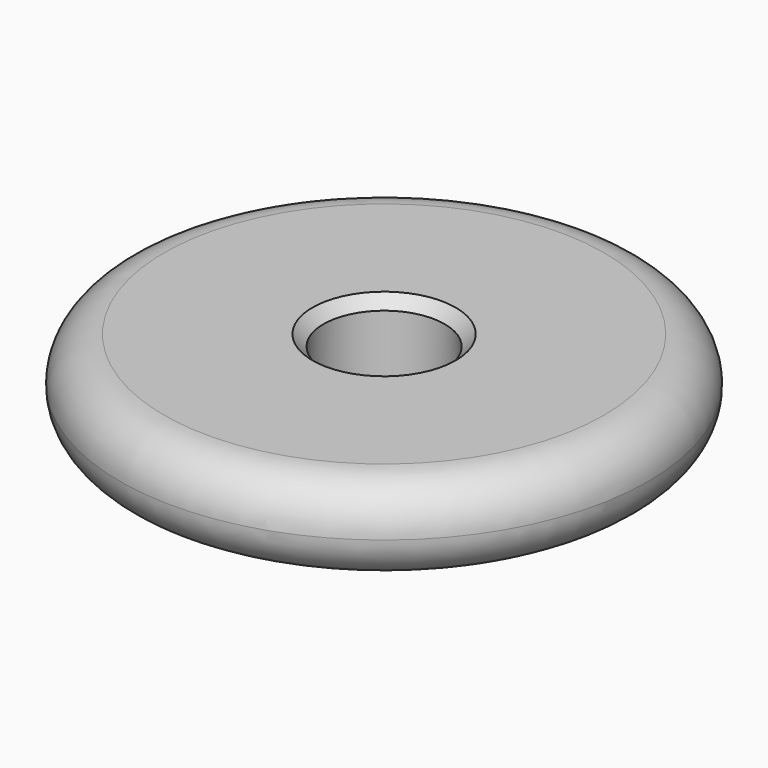
from build123d import *

# Parameters (mm, degrees)
F0_R     = 30.48
F0_R_2   = 6.9999987
F1_DEPTH = 10.16
F2_R     = 5.07999
F3_SIZE  = 1.27


# Not quite as in the source:
# - a fillet or chamfer is up to 0.001 mm smaller than in the source, because OpenCascade refuses the exact size


with BuildPart() as f1:
    # F0 (on Top) → F1 (new body)
    with BuildSketch(Plane.XY):
        Circle(F0_R)
        Circle(F0_R_2, mode=Mode.SUBTRACT)
    extrude(amount=F1_DEPTH)

    # F2 (radius 5.08 in the source; OpenCascade refuses exactly that, so slightly less here)
    f2_edges = [f1.edges().sort_by_distance(p)[0] for p in [
        (-30.48, 0, 10.16),
        (-30.48, 0, 0),
    ]]
    fillet(f2_edges, radius=F2_R)

    # F3
    f3_edges = [f1.edges().sort_by_distance(p)[0] for p in [
        (-6.999999, 0, 10.16),
        (-6.999999, 0, 0),
    ]]
    chamfer(f3_edges, length=F3_SIZE)


solid = f1.part
